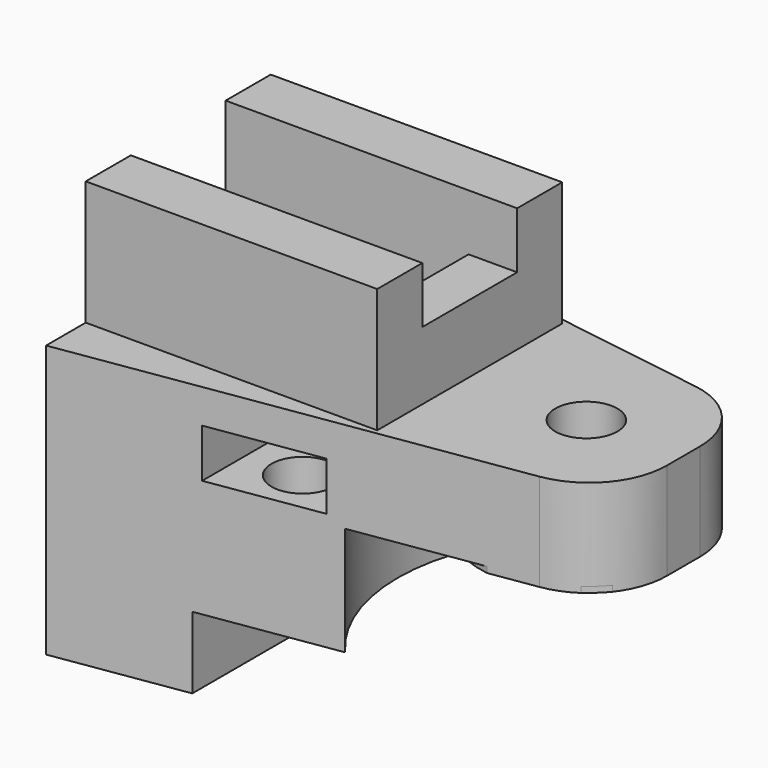
from build123d import *

# Parameters (mm, degrees)
F1_DEPTH        = 8
F1_DEPTH_BACK   = 6
F2_R            = 8.3
F2_R_2          = 2.95
F3_DEPTH        = 3
F3_DEPTH_BACK   = 3
F5_DEPTH        = 3.3
F5_DEPTH_BACK   = 3.3
F7_START        = -14
F6_R            = 3.15
F7_DEPTH        = 26
F9_DEPTH        = 5
F10_W           = 15
F10_H           = 2.9
F11_DEPTH       = 6.4
F12_W           = 1
F12_H           = 6.5
F13_DEPTH       = 3.5
F14_T4_DEPTH    = 31.8168298797
F16_D           = 3.2
F16_DEPTH       = 11
F16_CBORE_D     = 6.5
F16_CBORE_DEPTH = 2.5
F16_TIP         = 0.9613769904
F18_D           = 3.2
F18_CBORE_D     = 6.2
F18_CBORE_DEPTH = 2.6
F20_DEPTH       = 25
F20_DEPTH_BACK  = 25
F21_W           = 5.7
F21_H           = 2.5
F22_DEPTH       = 25
F22_DEPTH_BACK  = 25


# Not quite as in the source:
# - a fillet or chamfer that OpenCascade refuses, or shapes differently, is made with other operations: its cross-section is extruded or revolved along the edge and cut away or added


with BuildPart() as f1:
    # F0 (on Top) → F1 (new body, two sides)
    with BuildSketch(Plane.XY) as f1_sk:
        with BuildLine():
            Line((-21, -8.5), (1.608228737, -5.0218109635))
            ThreePointArc((1.608228737, -5.0218109635), (4.0358618997, -3.6728476468), (5, -1.0683241729))
            Line((5, -1.0683241729), (5, 1.0683241729))
            ThreePointArc((5, 1.0683241729), (4.0358618997, 3.6728476468), (1.608228737, 5.0218109635))
            Line((1.608228737, 5.0218109635), (-21, 8.5))
            Line((-21, 8.5), (-21, -8.5))
        make_face()
    extrude(amount=F1_DEPTH)
    extrude(f1_sk.sketch, amount=-F1_DEPTH_BACK)

    # F2 (on Top) → F3 (cut, two sides)
    with BuildSketch(Plane.XY) as f3_sk:
        Circle(F2_R)
        Circle(F2_R_2, mode=Mode.SUBTRACT)
    extrude(amount=-F3_DEPTH, mode=Mode.SUBTRACT)
    extrude(f3_sk.sketch, amount=F3_DEPTH_BACK, mode=Mode.SUBTRACT)

    # F4 (on Top) → F5 (cut, two sides)
    with BuildSketch(Plane.XY) as f5_sk:
        with BuildLine():
            ThreePointArc((5, -2.1685248442), (-5.45, 0), (5, 2.1685248442))
            Line((5, 2.1685248442), (5, 8.3120394609))
            ThreePointArc((5, 8.3120394609), (-9.7, 0), (5, -8.3120394609))
            Line((5, -8.3120394609), (5, -2.1685248442))
        make_face()
    extrude(amount=F5_DEPTH, mode=Mode.SUBTRACT)
    extrude(f5_sk.sketch, amount=-F5_DEPTH_BACK, mode=Mode.SUBTRACT)

    # F6 (on Right) → F7 (cut)
    with BuildSketch(Plane.YZ.offset(F7_START)):
        with Locations((0, 0.5)):
            Circle(F6_R)
    extrude(amount=-F7_DEPTH, mode=Mode.SUBTRACT)

    # F8 (on face) → F9 (cut)
    with BuildSketch(Plane(origin=(-21, 0, 0), x_dir=(0, -1, 0), z_dir=(-1, 0, 0))):
        Polygon((2.9444863729, 5.6), (-2.9444863729, 5.6), (-5.8889727457, 0.5), (-2.9444863729, -4.6), (2.9444863729, -4.6), (5.8889727457, 0.5), align=None)
    extrude(amount=-F9_DEPTH, mode=Mode.SUBTRACT)

    # F10 (on face) → F11 (join)
    with BuildSketch(Plane.XY.offset(8)):
        with Locations((-13.5, 4.5)):
            Rectangle(F10_W, F10_H)
        with Locations((-13.5, -4.5)):
            Rectangle(F10_W, F10_H)
    extrude(amount=F11_DEPTH)

    # F12 (on face) → F13 (join)
    with BuildSketch(Plane.XY.offset(8)):
        with Locations((-6.5, 0)):
            Rectangle(F12_W, F12_H)
    extrude(amount=F13_DEPTH)

    # F14: chamfer of 5 on 1 edges, made by hand


with BuildPart() as f14_tool2:
    # F14_s3 → F14_t4 (new body)
    with BuildSketch(Plane.XZ.offset(-15.9084149398)):
        Polygon((-7, 13), (-12, 8), (-7, 8), align=None)
    extrude(amount=F14_T4_DEPTH)

    split(bisect_by=Plane.XY.offset(11.5), keep=Keep.BOTTOM)

    split(bisect_by=Plane.XZ.offset(-5.95), keep=Keep.TOP)

    split(bisect_by=Plane.XZ.offset(5.95), keep=Keep.BOTTOM)


with BuildPart() as f1_1:
    add(f1.part)

    # F14_t1: union F14_tool2
    add(f14_tool2.part)

    # F16
    with Locations(Plane(origin=(0, 0, -6), x_dir=(1, 0, 0), z_dir=(0, 0, -1))):
        with Locations((-11, -4.5), (-11, 4.5)):
            CounterBoreHole(F16_D / 2, F16_CBORE_D / 2, F16_CBORE_DEPTH, depth=F16_DEPTH)
            with Locations((0, 0, -(F16_DEPTH + F16_TIP / 2))):  # 118° drill point
                Cone(0, F16_D / 2, F16_TIP, mode=Mode.SUBTRACT)

    # F18 (through all)
    with Locations(Plane(origin=(0, 0, -6), x_dir=(1, 0, 0), z_dir=(0, 0, -1))):
        with Locations((0, 0)):
            CounterBoreHole(F18_D / 2, F18_CBORE_D / 2, F18_CBORE_DEPTH)

    # F19 (on Front) → F20 (cut, two sides)
    with BuildSketch(Plane.XZ) as f20_sk:
        Polygon((9.8263500258, -7.5822613659), (9.9938229204, 3), (-6.1094067059, 3), (-6.1094067059, -2.3), (-14.3, -2.3), (-14.3, -7.5822613659), align=None)
    extrude(amount=-F20_DEPTH, mode=Mode.SUBTRACT)
    extrude(f20_sk.sketch, amount=F20_DEPTH_BACK, mode=Mode.SUBTRACT)

    # F21 (on Front) → F22 (cut, two sides)
    with BuildSketch(Plane.XZ) as f22_sk:
        with Locations((-11, 5)):
            Rectangle(F21_W, F21_H)
    extrude(amount=-F22_DEPTH, mode=Mode.SUBTRACT)
    extrude(f22_sk.sketch, amount=F22_DEPTH_BACK, mode=Mode.SUBTRACT)


solid = f1_1.part
